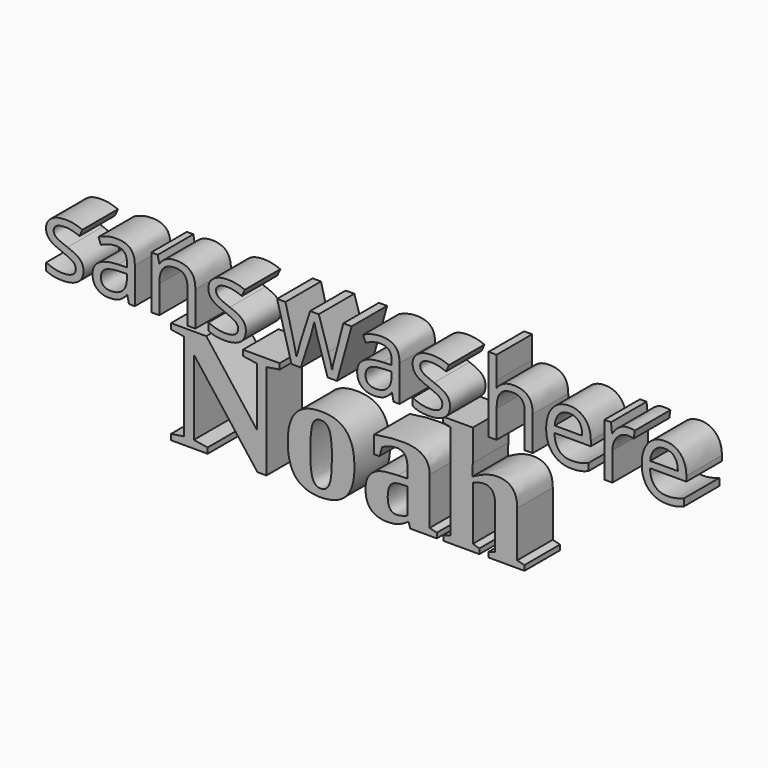
from build123d import *

# Parameters (mm, degrees)
F0_TEXT_SIZE = 180.1172995733
F1_DEPTH     = 50.8
F2_TEXT_SIZE = 112.7401935971
F3_DEPTH     = 50.8


# Not quite as in the source:
# - Text() gives the source's letters only with a copy of the font that has no kerning and outlines rounded to 1/6400 em; it was checked with that copy


with BuildPart() as f1:
    # F0 (on Front) → F1 (new body)
    with BuildSketch(Plane.XZ):
        with Locations((-197.890162468, -63.6790134013)):
            Text('Noah', F0_TEXT_SIZE, font='Tinos', font_style=FontStyle.BOLD, text_align=(TextAlign.LEFT, TextAlign.BOTTOM))
    extrude(amount=F1_DEPTH)


with BuildPart() as f3:
    # F2 (on face) → F3 (new body)
    with BuildSketch(Plane.XZ.offset(50.8)):
        with Locations((-302.4969995022, 91.6599966586)):
            Text('sans was here', F2_TEXT_SIZE, font='Open Sans', text_align=(TextAlign.LEFT, TextAlign.BOTTOM))
    extrude(amount=F3_DEPTH)


solid = Compound([f1.part, f3.part])
